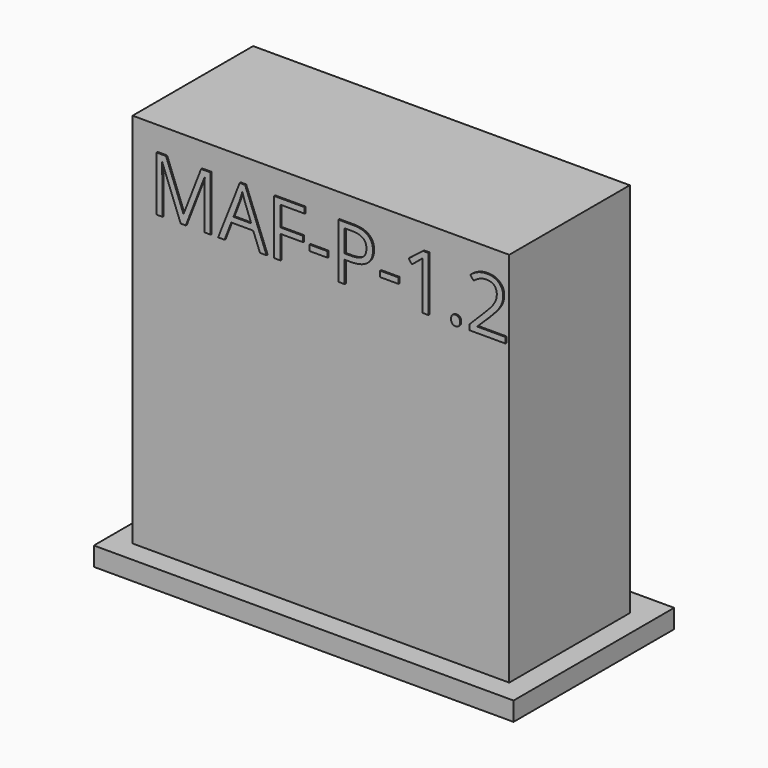
from build123d import *

# Parameters (mm, degrees)
F0_W         = 1778
F0_H         = 711.2
F1_DEPTH     = 1778
F2_TEXT_SIZE = 361.7371122042
F3_DEPTH     = 6.35
F4_DEPTH     = 88.9
F5_W         = 711.2
F5_H         = 88.9
F6_DEPTH     = 101.6
F7_W         = 1879.6
F7_H         = 88.9
F8_DEPTH     = 101.6
F10_DEPTH    = 101.6
F12_DEPTH    = 134.96798


# Not quite as in the source:
# - Text() gives the source's letters only with a copy of the font that has no kerning and outlines rounded to 1/6400 em; it was checked with that copy


with BuildPart() as f1:
    # F0 (on Top) → F1 (new body)
    with BuildSketch(Plane.XY):
        with Locations((889, 355.6)):
            Rectangle(F0_W, F0_H)
    extrude(amount=F1_DEPTH)

    # F2 (on face) → F3 (join)
    with BuildSketch(Plane.XZ):
        with Locations((82.2138339281, 1407.5598716736)):
            Text('MAF-P-1.2', F2_TEXT_SIZE, font='Open Sans', text_align=(TextAlign.LEFT, TextAlign.BOTTOM))
    extrude(amount=F3_DEPTH)

    # F4 (add): a face of the model
    f4_faces = [f1.faces().sort_by_distance(p)[0] for p in [
        (889, 355.6, 0),
    ]]
    extrude(f4_faces, amount=F4_DEPTH)

    # F5 (on face) → F6 (join)
    with BuildSketch(Plane(origin=(0, 0, 0), x_dir=(0, -1, 0), z_dir=(-1, 0, 0))):
        with Locations((-355.6, -44.45)):
            Rectangle(F5_W, F5_H)
    extrude(amount=F6_DEPTH)

    # F7 (on face) → F8 (join)
    with BuildSketch(Plane.XZ):
        with Locations((838.2, -44.45)):
            Rectangle(F7_W, F7_H)
    extrude(amount=F8_DEPTH)

    # F9 (on face) → F10 (join)
    with BuildSketch(Plane.YZ.offset(1778)):
        Polygon((-101.6, 0), (-101.6, -88.9), (711.2, -88.9), (711.2, 0), (0, 0), align=None)
    extrude(amount=F10_DEPTH)

    # F11 (on face) → F12 (join)
    with BuildSketch(Plane(origin=(0, 711.2, 0), x_dir=(-1, 0, 0), z_dir=(0, 1, 0))):
        Polygon((-1879.6, -88.9), (101.6, -88.9), (101.6, 0), (0, 0), (-1778, 0), (-1879.6, 0), align=None)
    extrude(amount=F12_DEPTH)


solid = f1.part
